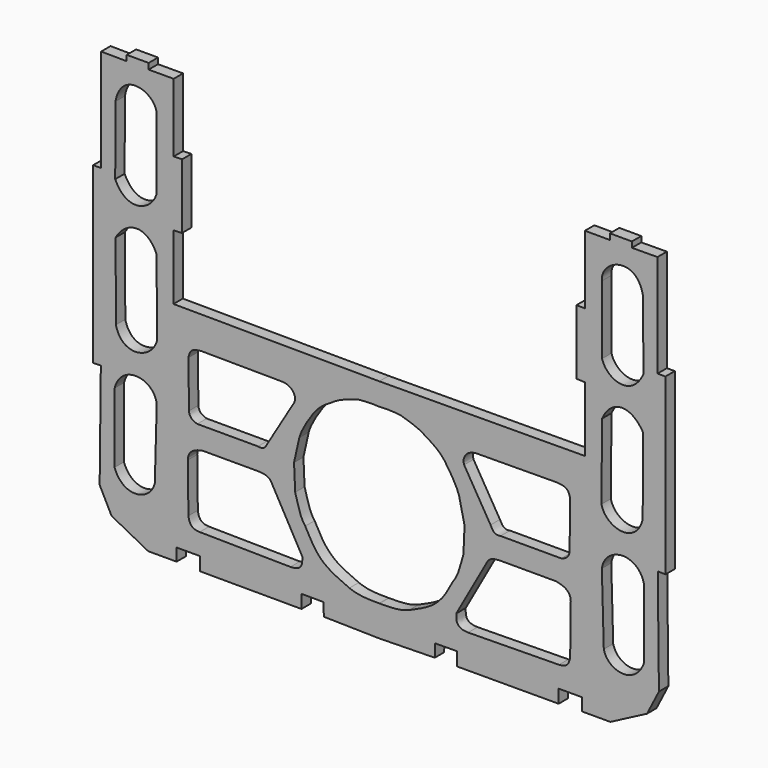
from build123d import *

# Parameters (mm, degrees)
F1_DEPTH = 4


# Not quite as in the source:
# - ends of sketch curves that miss each other by under 0.0002 mm in the source are joined


with BuildPart() as f1:
    # F0 (on Front) → F1 (new body)
    with BuildSketch(Plane.XZ):
        with BuildLine():
            Line((0, -62.5768265655), (0, -73.0655565858))
            Line((0, -73.0655565858), (18.8595041584, -72.6991555655))
            Line((18.8595041584, -72.6991555655), (18.9268171584, -68.3466805655))
            Line((18.9268171584, -68.3466805655), (26.3961031584, -68.2965805655))
            Line((26.3961031584, -68.2965805655), (26.4462181584, -72.8495015655))
            Line((26.4462181584, -72.8495015655), (60.9480091584, -72.7822265655))
            Line((60.9480091584, -72.7822265655), (60.9480091584, -68.2464965655))
            Line((60.9480091584, -68.2464965655), (68.8855091584, -68.2464965655))
            Line((68.8855091584, -68.2464965655), (68.8855091584, -72.4987415655))
            Line((68.8855091584, -72.4987415655), (78.5239021584, -72.4987415655))
            Line((78.5239021584, -72.4987415655), (90.9971141584, -65.9786385655))
            Line((90.9971141584, -65.9786385655), (95.0367341584, -58.0411565655))
            Line((95.0367341584, -58.0411565655), (94.6358591584, -22.1866785655))
            Line((94.6358591584, -22.1866785655), (97.2417351584, -22.2869085655))
            Line((97.2417351584, -22.2869085655), (97.2337091584, 36.9253744345))
            Line((97.2337091584, 36.9253744345), (94.5406391584, 36.9253744345))
            Line((94.5406391584, 36.9253744345), (94.5406391584, 71.7936764345))
            Line((94.5406391584, 71.7936764345), (85.8443141584, 71.7270764345))
            Line((85.8443141584, 71.7270764345), (85.8356901584, 73.6276884345))
            Line((85.8356901584, 73.6276884345), (78.3821291584, 73.6363144345))
            Line((78.3821291584, 73.6363144345), (78.3900041584, 71.6268764345))
            Line((78.3900041584, 71.6268764345), (69.8776841584, 71.6519264345))
            Line((69.8776841584, 71.6519264345), (69.8776841584, 48.4063814345))
            Line((69.8776841584, 48.4063814345), (67.0428631584, 48.4772564345))
            Line((67.0428631584, 48.4772564345), (67.0428621584, 26.4365264345))
            Line((67.0428621584, 26.4365264345), (69.9485551584, 26.2947834345))
            Line((69.9485551584, 26.2947834345), (69.9485551584, 4.2540534345))
            Line((69.9485551584, 4.2540534345), (0, 3.8812716957))
            Line((0, 3.8812716957), (0, -3.7450785655))
            Line((0, -3.7450785655), (0.1226601584, -3.7450785655))
            add(Edge.make_bspline(
                [(0.1226601584, -3.7450785655), (2.5280861584, -3.5204685655), (4.9335121584, -3.6365465655), (7.3389371584, -3.9455235655)],
                knots=[0, 0, 0, 0, 1, 1, 1, 1], degree=3))
            add(Edge.make_bspline(
                [(7.3389371584, -3.9455235655), (10.2033821584, -4.8083315655), (13.0099951584, -5.6959265655), (14.9561191584, -6.9523035655)],
                knots=[0, 0, 0, 0, 1, 1, 1, 1], degree=3))
            add(Edge.make_bspline(
                [(14.9561191584, -6.9523035655), (17.3970001584, -8.5046165655), (19.8799371584, -9.6883565655), (22.1602361584, -12.6479915655)],
                knots=[0, 0, 0, 0, 1, 1, 1, 1], degree=3))
            add(Edge.make_bspline(
                [(22.1602361584, -12.6479915655), (24.2064201584, -15.6312885655), (26.2339181584, -18.6177065655), (27.1715391584, -21.7857665655)],
                knots=[0, 0, 0, 0, 1, 1, 1, 1], degree=3))
            Line((27.1715391584, -21.7857665655), (28.9756101584, -29.8646385655))
            Line((28.9756101584, -29.8646385655), (28.5868641584, -38.6237465655))
            add(Edge.make_bspline(
                [(28.5868641584, -38.6237465655), (27.7046781584, -41.1933815655), (27.2918321584, -44.8986885655), (25.1791781584, -47.6441085655)],
                knots=[0, 0, 0, 0, 1, 1, 1, 1], degree=3))
            add(Edge.make_bspline(
                [(25.1791781584, -47.6441085655), (20.8753181584, -55.9524065655), (18.9745221584, -57.4683285655), (10.1452671584, -61.2748485655)],
                knots=[0, 0, 0, 0, 1, 1, 1, 1], degree=3))
            add(Edge.make_bspline(
                [(10.1452671584, -61.2748485655), (6.9815371584, -62.5751165655), (3.4302711584, -62.5658085655), (0.0823671584, -62.5768635655)],
                knots=[0, 0, 0, 0, 1, 1, 1, 1], degree=3))
            Line((0.0823671584, -62.5768635655), (0, -62.5768265655))
        make_face()
        with BuildLine():
            add(Edge.make_bspline(
                [(36.8054091584, -38.0223665655), (37.7203301584, -36.6333885655), (39.3608411584, -36.5141985655), (41.0149061584, -36.4187315655)],
                knots=[0, 0, 0, 0, 1, 1, 1, 1], degree=3))
            Line((41.0149061584, -36.4187315655), (60.2583101584, -36.4187315655))
            add(Edge.make_bspline(
                [(60.2583101584, -36.4187315655), (62.7480351584, -37.0026135655), (64.9984411584, -37.8258055655), (65.0691611584, -40.8286935655)],
                knots=[0, 0, 0, 0, 1, 1, 1, 1], degree=3))
            Line((65.0691611584, -40.8286935655), (64.8687101584, -57.4662285655))
            add(Edge.make_bspline(
                [(64.8687101584, -57.4662285655), (64.4598401584, -60.7591105655), (62.7602801584, -60.9174655655), (61.0601191584, -61.0743585655)],
                knots=[0, 0, 0, 0, 1, 1, 1, 1], degree=3))
            Line((61.0601191584, -61.0743585655), (30.1904901584, -61.4752555655))
            add(Edge.make_bspline(
                [(30.1904901584, -61.4752555655), (26.0151861584, -61.3630405655), (26.1180031584, -59.2047655655), (26.1814461584, -57.0653235655)],
                knots=[0, 0, 0, 0, 1, 1, 1, 1], degree=3))
            Line((26.1814461584, -57.0653235655), (36.8054091584, -38.0223665655))
        make_face(mode=Mode.SUBTRACT)
        with BuildLine():
            add(Edge.make_bspline(
                [(28.8374371584, -11.7631335655), (28.1155241584, -9.8636235655), (29.3390181584, -6.8925585655), (33.5981751584, -6.9522735655)],
                knots=[0, 0, 0, 0, 1, 1, 1, 1], degree=3))
            Line((33.5981751584, -6.9522735655), (60.4587621584, -6.7518355655))
            add(Edge.make_bspline(
                [(60.4587621584, -6.7518355655), (62.2697401584, -7.0595985655), (64.3212711584, -6.7831865655), (64.8687101584, -10.1595215655)],
                knots=[0, 0, 0, 0, 1, 1, 1, 1], degree=3))
            Line((64.8687101584, -10.1595215655), (64.6682581584, -25.9952315655))
            add(Edge.make_bspline(
                [(64.6682581584, -25.9952315655), (64.5461211584, -27.9269835655), (63.2897931584, -28.5625185655), (61.8619271584, -29.0020115655)],
                knots=[0, 0, 0, 0, 1, 1, 1, 1], degree=3))
            Line((61.8619271584, -29.0020115655), (41.2153571584, -29.0020115655))
            add(Edge.make_bspline(
                [(41.2153571584, -29.0020115655), (38.8857901584, -29.4606885655), (38.5168061584, -27.9587835655), (37.8076711584, -26.7970335655)],
                knots=[0, 0, 0, 0, 1, 1, 1, 1], degree=3))
            Line((37.8076711584, -26.7970335655), (28.8374371584, -11.7631335655))
        make_face(mode=Mode.SUBTRACT)
        with BuildLine():
            add(Edge.make_bspline(
                [(75.6344151584, -27.5401405655), (76.7086701584, -20.0264385655), (87.7931151584, -18.8621605655), (89.9252301584, -27.3983985655)],
                knots=[0, 0, 0, 0, 1, 1, 1, 1], degree=3))
            Line((89.9252301584, -27.3983985655), (89.9718051584, -51.1570035655))
            add(Edge.make_bspline(
                [(89.9718051584, -51.1570035655), (86.9677921584, -59.3849455655), (77.6966521584, -57.5675315655), (76.2945051584, -51.4526535655)],
                knots=[0, 0, 0, 0, 1, 1, 1, 1], degree=3))
            Line((76.2945051584, -51.4526535655), (75.6344151584, -27.5401405655))
        make_face(mode=Mode.SUBTRACT)
        with BuildLine():
            add(Edge.make_bspline(
                [(75.7174401584, 17.3510644345), (78.9392901584, 24.7262494345), (85.8315491584, 24.2653064345), (89.5951921584, 17.7762844345)],
                knots=[0, 0, 0, 0, 1, 1, 1, 1], degree=3))
            Line((89.5951921584, 17.7762844345), (89.5243171584, -8.3554485655))
            add(Edge.make_bspline(
                [(89.5243171584, -8.3554485655), (87.2297001584, -17.4540505655), (76.9894851584, -14.8237105655), (75.4926641584, -8.3554485655)],
                knots=[0, 0, 0, 0, 1, 1, 1, 1], degree=3))
            Line((75.4926641584, -8.3554485655), (75.7174401584, 17.3510644345))
        make_face(mode=Mode.SUBTRACT)
        with BuildLine():
            add(Edge.make_bspline(
                [(75.6465721584, 58.5247134345), (75.1134871584, 65.2343494345), (87.6475471584, 69.7689614345), (89.6417451584, 58.4538384345)],
                knots=[0, 0, 0, 0, 1, 1, 1, 1], degree=3))
            Line((89.6417451584, 58.4538384345), (89.7490921584, 35.1548344345))
            add(Edge.make_bspline(
                [(89.7490921584, 35.1548344345), (85.7240821584, 26.3078794345), (77.2700671584, 29.6706164345), (75.7174401584, 35.2722614345)],
                knots=[0, 0, 0, 0, 1, 1, 1, 1], degree=3))
            Line((75.7174401584, 35.2722614345), (75.6465721584, 58.5247134345))
        make_face(mode=Mode.SUBTRACT)
    extrude(amount=F1_DEPTH)

    # F2: F1 across plane


with BuildPart() as f1_1:
    add(f1.part)
    add(f1.part.mirror(Plane.YZ))


solid = f1_1.part
